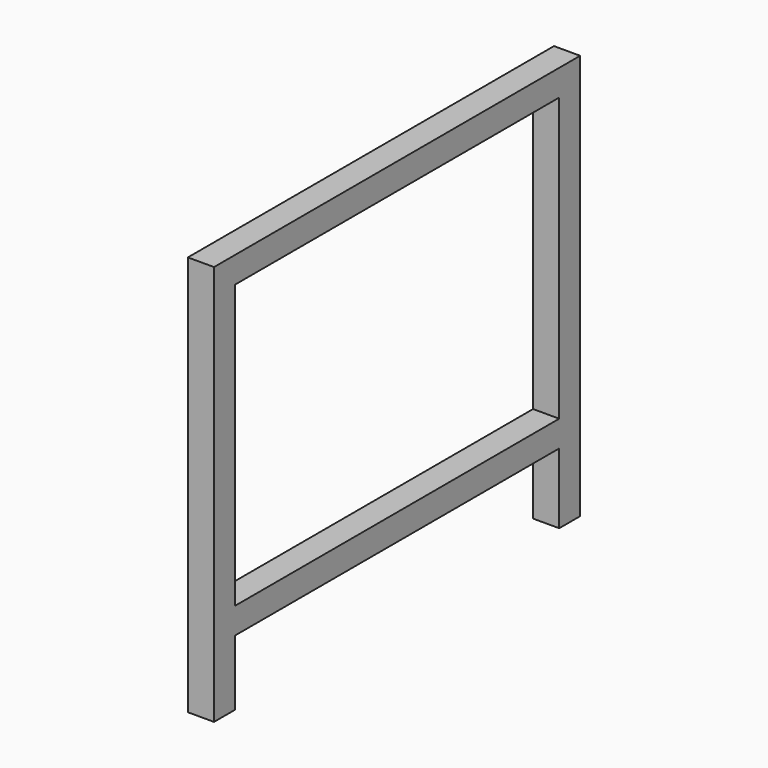
from build123d import *

# Parameters (mm, degrees)
F0_W     = 620
F0_H     = 432.4773087313
F1_DEPTH = 40


# Not quite as in the source:
# - a feature names something its author has since deleted; it is built from what else it names


with BuildPart() as f1:
    # F0 (on Right) → F1 (new body)
    with BuildSketch(Plane.YZ):
        Polygon((406.8596840377, -620), (406.8596840377, 0), (-293.1403159623, 0), (-293.1403159623, -612.4773087313), (-253.1403159623, -612.4773087313), (-253.1403159623, -512.4773087313), (366.8596840377, -512.4773087313), (366.8596840377, -620), align=None)
        with Locations((56.8596840377, -256.2386543657)):
            Rectangle(F0_W, F0_H, mode=Mode.SUBTRACT)
    extrude(amount=F1_DEPTH)


solid = f1.part
